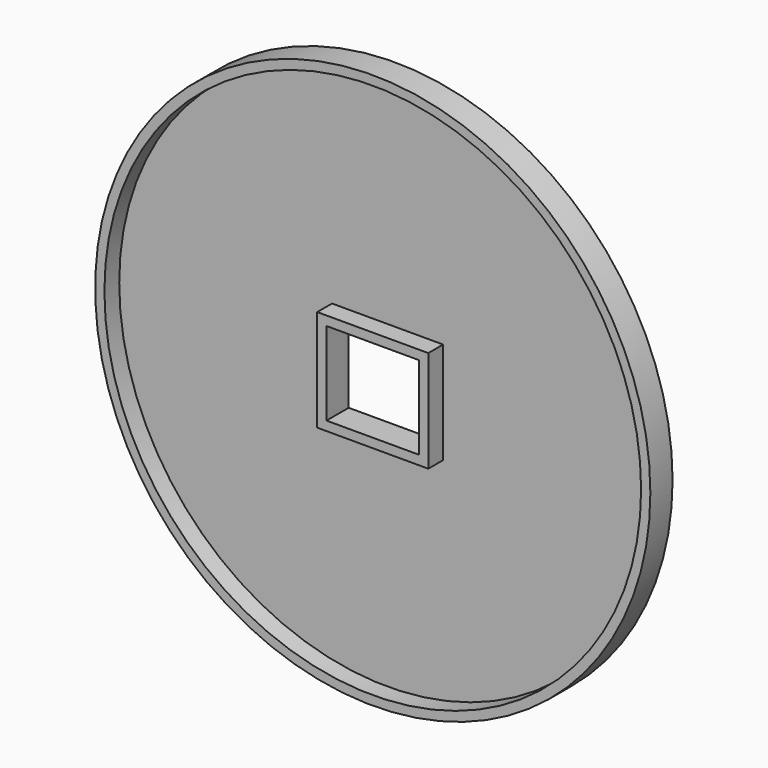
from build123d import *

# Parameters (mm, degrees)
F0_R     = 76.2
F0_W     = 25.4
F0_H     = 22.86
F1_DEPTH = 7.62
F3_T     = -2.54


# Not quite as in the source:
# - the program builds the solid bodies; features that only make, move or delete a surface that nothing else refers to are left out


with BuildPart() as f1:
    # F0 (on Front) → F1 (new body)
    with BuildSketch(Plane.XZ):
        with Locations((40.9205045223, 25.0884863067)):
            Circle(F0_R)
        with Locations((40.9205045223, 25.0884863067)):
            Rectangle(F0_W, F0_H, mode=Mode.SUBTRACT)
    extrude(amount=F1_DEPTH)

    # F3
    f3_openings = [f1.faces().sort_by_distance(p)[0] for p in [
        (-33.124234, -7.62, 25.088486),
    ]]
    offset(amount=F3_T, openings=f3_openings, kind=Kind.INTERSECTION)


solid = f1.part
